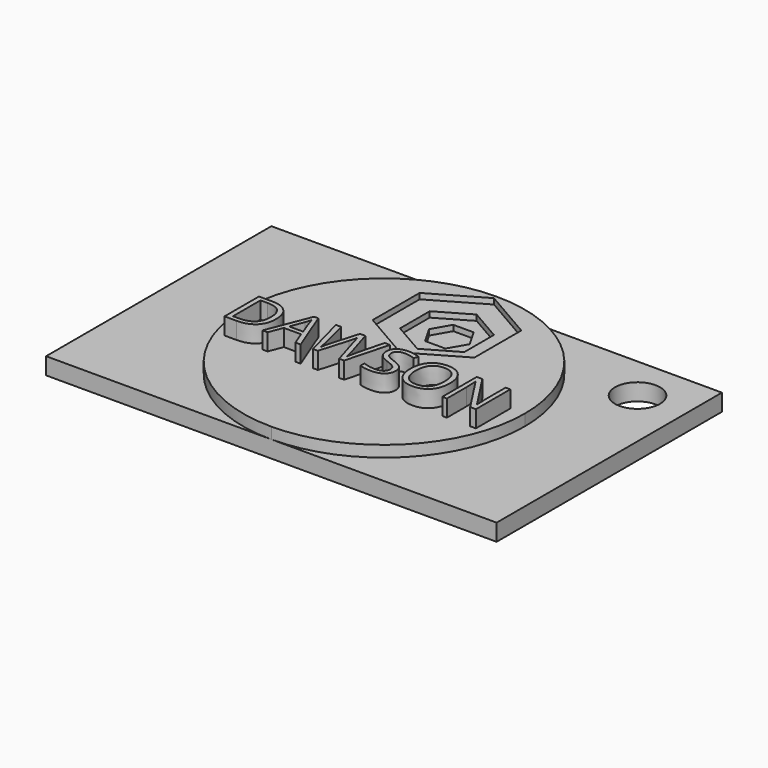
from build123d import *

# Parameters (mm, degrees)
F1_W         = 80
F1_H         = 50
F2_DEPTH     = 3
F4_DEPTH     = 2
F5_R         = 4
F6_DEPTH     = 3
F6_FACE_R    = 4
F7_DEPTH     = 3
F8_TEXT_SIZE = 10.69444568
F9_DEPTH     = 3
F11_DEPTH    = 1
F13_DEPTH    = 1
F15_DEPTH    = 1


# Not quite as in the source:
# - Text() gives the source's letters only with a copy of the font that has no kerning and outlines rounded to 1/6400 em; it was checked with that copy


with BuildPart() as f2:
    # F1 (on face) → F2 (new body)
    with BuildSketch(Plane.XY):
        Rectangle(F1_W, F1_H)
    extrude(amount=F2_DEPTH)

    # F3 (on face) → F4 (join)
    with BuildSketch(Plane.XY.offset(3)):
        with BuildLine():
            ThreePointArc((3.65e-08, -25), (17.6776695426, -17.6776695168), (25, 0))
            ThreePointArc((25, 0), (17.6776695297, 17.6776695297), (0, 25))
            ThreePointArc((0, 25), (-25, -1.82e-08), (3.65e-08, -25))
        make_face()
    extrude(amount=F4_DEPTH)

    # F5 (on face) → F6 (cut)
    with BuildSketch(Plane.XY.offset(5)):
        with Locations((31.4125008881, 17)):
            Circle(F5_R)
    extrude(amount=-F6_DEPTH, mode=Mode.SUBTRACT)

    # F5 (on face) + F6_face (on face) → F7 (cut)
    with BuildSketch(Plane.XY.offset(5)):
        with Locations((31.4125008881, 17)):
            Circle(F5_R)
    with BuildSketch(Plane(origin=(31.4125008881, 17, 2), x_dir=(1, 0, 0), z_dir=(0, 0, 1))):
        Circle(F6_FACE_R)
    extrude(amount=-F7_DEPTH, mode=Mode.SUBTRACT)

    # F8 (on face) → F9 (join)
    with BuildSketch(Plane.XY.offset(5)):
        with Locations((-23.2034418732, -7.7000008896)):
            Text('DAWSON', F8_TEXT_SIZE, font='Open Sans', text_align=(TextAlign.LEFT, TextAlign.BOTTOM))
    extrude(amount=F9_DEPTH)

    # F10 (on face) → F11 (cut)
    with BuildSketch(Plane.XY.offset(5)):
        Polygon((-9.028442204, 19.1928746339), (-9.028442204, 8.7677275602), (0, 3.5551540234), (9.028442204, 8.7677275602), (9.028442204, 19.1928746339), (0, 24.4054481707), align=None)
    extrude(amount=-F11_DEPTH, mode=Mode.SUBTRACT)

    # F12 (on face) → F13 (cut)
    with BuildSketch(Plane.XY.offset(4)):
        Polygon((-5.703441333, 17.273184486), (-5.703441333, 10.6874177081), (0, 7.3945343192), (5.703441333, 10.6874177081), (5.703441333, 17.273184486), (0, 20.5660678749), align=None)
    extrude(amount=-F13_DEPTH, mode=Mode.SUBTRACT)

    # F14 (on face) → F15 (cut)
    with BuildSketch(Plane.XY.offset(3)):
        Polygon((-3.6106961211, 14.5053016022), (-1.8053480605, 11.378347036), (1.8053480605, 11.378347036), (3.6106961211, 14.5053016022), (1.8053480605, 17.6322561684), (-1.8053480605, 17.6322561684), align=None)
    extrude(amount=-F15_DEPTH, mode=Mode.SUBTRACT)


solid = f2.part
